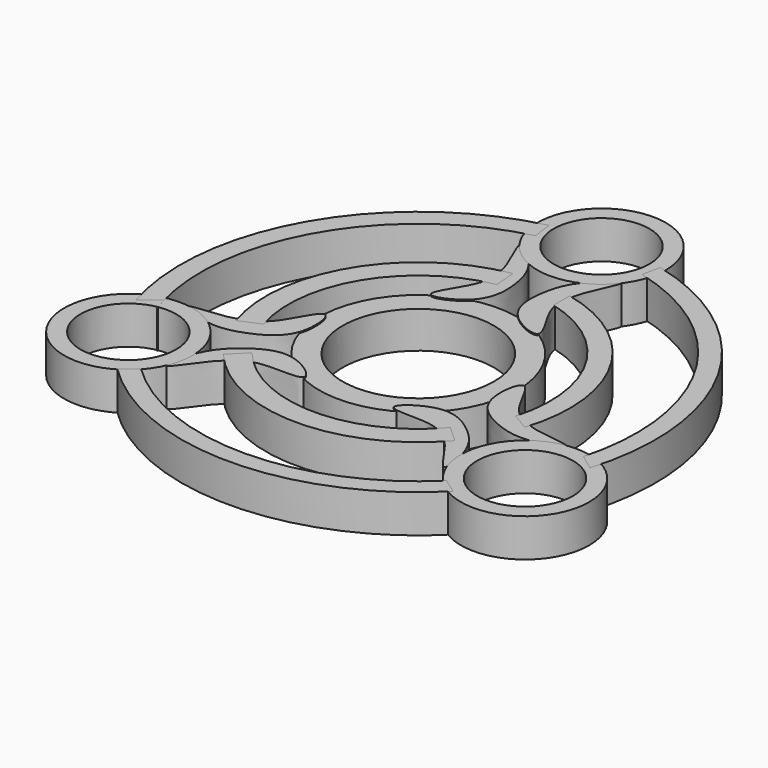
from build123d import *

# Parameters (mm, degrees)
F0_R      = 19.8316168412
F1_DEPTH  = 7.366
F2_R      = 15.1327699345
F3_DEPTH  = 8.89
F4_R      = 12.8405806387
F4_R_2    = 9.5708012392
F5_DEPTH  = 7.62
F7_DEPTH  = 7.62
F8_DEPTH  = 7.62
F10_DEPTH = 7.62
F12_DEPTH = 7.62


# Not quite as in the source:
# - a feature of the source that left no trace in its solid (it failed there, or was rolled back) is left out
# - a feature names something its author has since deleted; it is built from what else it names


with BuildPart() as f1:
    # F0 (on Top) → F1 (new body)
    with BuildSketch(Plane.XY):
        Circle(F0_R)
    extrude(amount=F1_DEPTH)

    # F2 (on Top) → F3 (cut)
    with BuildSketch(Plane.XY):
        Circle(F2_R)
    extrude(amount=F3_DEPTH, mode=Mode.SUBTRACT)


with BuildPart() as f5:
    # F4 (on Top) → F5 (new body)
    with BuildSketch(Plane.XY):
        with Locations((0, 45.8028241992)):
            Circle(F4_R)
        with Locations((0, 45.8028241992)):
            Circle(F4_R_2, mode=Mode.SUBTRACT)
    extrude(amount=F5_DEPTH)


with BuildPart() as f7:
    # F6 (on Top) → F7 (new body)
    with BuildSketch(Plane.XY):
        with BuildLine():
            add(Edge.make_bspline(
                [(-10.1461960003, 38.2656529546), (-10.5971686857, 37.8400995519), (-7.5929666267, 32.2725156605), (-6.9075768698, 28.4550696213), (-6.4560361932, 23.7178665225), (-14.0221319892, 14.0519491431), (-2.2026089144, 18.9490453351), (-2.2410472149, 27.8294457935), (-4.2881589957, 34.1102219148), (-9.6911539418, 38.6950463582), (-10.1461960003, 38.2656529546)],
                knots=[0, 0, 0, 0, 0.1196064646, 0.2243344987, 0.3343048571, 0.4708784974, 0.6015443046, 0.7437811682, 0.8793142609, 1, 1, 1, 1], degree=3))
        make_face()
    extrude(amount=F7_DEPTH)


with BuildPart() as f7b:
    # F6 (on Top) → F7, piece 2 (new body)
    with BuildSketch(Plane.XY):
        with BuildLine():
            add(Edge.make_bspline(
                [(10.1461960003, 38.2656529546), (10.5971686857, 37.8400995519), (7.5929666267, 32.2725156605), (6.9075768698, 28.4550696213), (6.4560361932, 23.7178665225), (14.0221319892, 14.0519491431), (2.2026089144, 18.9490453351), (2.2410472149, 27.8294457935), (4.2881589957, 34.1102219148), (9.6911539418, 38.6950463582), (10.1461960003, 38.2656529546)],
                knots=[0, 0, 0, 0, 0.1196064646, 0.2243344987, 0.3343048571, 0.4708784974, 0.6015443046, 0.7437811682, 0.8793142609, 1, 1, 1, 1], degree=3))
        make_face()
    extrude(amount=F7_DEPTH)


with BuildPart() as f7c:
    # F6 (on Top) → F7, piece 3 (new body)
    with BuildSketch(Plane.XY):
        with BuildLine():
            add(Edge.make_bspline(
                [(38.0458038622, -10.4497247993), (37.9192240951, -9.8427242852), (31.6027522683, -9.488599928), (27.9911987139, -8.074621744), (23.7183170825, -5.9799941528), (19.4420127466, 5.5260471128), (17.4286413404, -7.1083904453), (25.0157130247, -11.7235104937), (31.4389658818, -13.2664421394), (38.1735258277, -11.0622026108), (38.0458038622, -10.4497247993)],
                knots=[0, 0, 0, 0, 0.1196064646, 0.2243344987, 0.3343048571, 0.4708784974, 0.6015443046, 0.7437811682, 0.8793142609, 1, 1, 1, 1], degree=3))
        make_face()
    extrude(amount=F7_DEPTH)


with BuildPart() as f7d:
    # F6 (on Top) → F7, piece 4 (new body)
    with BuildSketch(Plane.XY):
        with BuildLine():
            add(Edge.make_bspline(
                [(27.4250593609, -27.7407906815), (26.8264144307, -27.9023342025), (23.6546544249, -22.4284727808), (20.7605470435, -19.8464588679), (16.9603251319, -16.9823192757), (4.7640505609, -18.3703578085), (15.1230140377, -10.862058899), (22.6698496209, -15.542685191), (26.9502450772, -20.5742883219), (28.0291061914, -27.577789465), (27.4250593609, -27.7407906815)],
                knots=[0, 0, 0, 0, 0.1196064646, 0.2243344987, 0.3343048571, 0.4708784974, 0.6015443046, 0.7437811682, 0.8793142609, 1, 1, 1, 1], degree=3))
        make_face()
    extrude(amount=F7_DEPTH)


with BuildPart() as f7e:
    # F6 (on Top) → F7, piece 5 (new body)
    with BuildSketch(Plane.XY):
        with BuildLine():
            add(Edge.make_bspline(
                [(-27.82798931, -28.063647449), (-27.2341608386, -28.2420845754), (-23.9086099711, -22.860269656), (-20.9425206648, -20.361276337), (-17.0626884028, -17.6059390074), (-4.9106288404, -19.338917014), (-15.0527396932, -11.540182227), (-22.729139541, -16.0051430533), (-27.1503526326, -20.9134717024), (-28.4271762203, -27.8836001869), (-27.82798931, -28.063647449)],
                knots=[0, 0, 0, 0, 0.1196064646, 0.2243344987, 0.3343048571, 0.4708784974, 0.6015443046, 0.7437811682, 0.8793142609, 1, 1, 1, 1], degree=3))
        make_face()
    extrude(amount=F7_DEPTH)


with BuildPart() as f7f:
    # F6 (on Top) → F7, piece 6 (new body)
    with BuildSketch(Plane.XY):
        with BuildLine():
            add(Edge.make_bspline(
                [(-37.9546495422, -10.4786559606), (-37.8109254408, -9.8754848039), (-31.4869568886, -9.700435813), (-27.8367974939, -8.3893333095), (-23.5062939642, -6.416588683), (-18.9057622264, 4.9636956767), (-17.2511076431, -7.722706297), (-24.9658717812, -12.1210473589), (-31.4302550876, -13.48140165), (-38.0996705446, -11.0872698603), (-37.9546495422, -10.4786559606)],
                knots=[0, 0, 0, 0, 0.1196064646, 0.2243344987, 0.3343048571, 0.4708784974, 0.6015443046, 0.7437811682, 0.8793142609, 1, 1, 1, 1], degree=3))
        make_face()
    extrude(amount=F7_DEPTH)


with BuildPart() as f8:
    # F4 (on Top) → F8 (new body)
    with BuildSketch(Plane.XY):
        with Locations((0, 45.8028241992)):
            Circle(F4_R)
        with Locations((0, 45.8028241992)):
            Circle(F4_R_2, mode=Mode.SUBTRACT)
    extrude(amount=F8_DEPTH)


with BuildPart() as f8b:
    # F4 (on Top) → F8, piece 2 (new body)
    with BuildSketch(Plane.XY):
        with Locations((-39.6664093216, -22.9014120996)):
            Circle(F4_R)
        with Locations((-39.6664093216, -22.9014120996)):
            Circle(F4_R_2, mode=Mode.SUBTRACT)
    extrude(amount=F8_DEPTH)


with BuildPart() as f8c:
    # F4 (on Top) → F8, piece 3 (new body)
    with BuildSketch(Plane.XY):
        with Locations((39.6664093216, -22.9014120996)):
            Circle(F4_R)
        with Locations((39.6664093216, -22.9014120996)):
            Circle(F4_R_2, mode=Mode.SUBTRACT)
    extrude(amount=F8_DEPTH)


with BuildPart() as f10:
    # F9 (on Top) → F10 (new body)
    with BuildSketch(Plane.XY):
        with BuildLine():
            Line((-4.7045984098, 25.5188748579), (-5.0730993971, 30.0037506968))
            ThreePointArc((-5.0730993971, 30.0037506968), (-26.0401835333, 15.7438951635), (-28.9256811899, -9.4480876938))
            Line((-28.9256811899, -9.4480876938), (-24.7857067734, -7.6821194962))
            ThreePointArc((-24.7857067734, -7.6821194962), (-22.2035139443, 13.4294522873), (-4.7045984098, 25.5188748579))
        make_face()
    extrude(amount=F10_DEPTH)


with BuildPart() as f10b:
    # F9 (on Top) → F10, piece 2 (new body)
    with BuildSketch(Plane.XY):
        with BuildLine():
            Line((-20.147446543, -16.378859058), (-23.336250335, -19.56766285))
            ThreePointArc((-23.336250335, -19.56766285), (-0.1568800839, -30.4540538804), (23.133416665, -19.8070452747))
            Line((23.133416665, -19.8070452747), (19.8330628805, -16.7581694413))
            ThreePointArc((19.8330628805, -16.7581694413), (-0.2463297861, -25.9639355237), (-20.147446543, -16.378859058))
        make_face()
    extrude(amount=F10_DEPTH)


with BuildPart() as f10c:
    # F9 (on Top) → F10, piece 3 (new body)
    with BuildSketch(Plane.XY):
        with BuildLine():
            Line((25.3654867411, -7.392228581), (28.8441870362, -9.4214677811))
            ThreePointArc((28.8441870362, -9.4214677811), (26.3563547864, 15.036413911), (6.5683197142, 29.6244553884))
            Line((6.5683197142, 29.6244553884), (6.5683197142, 25.5912121076))
            ThreePointArc((6.5683197142, 25.5912121076), (22.9547127753, 13.081824124), (25.3654867411, -7.392228581))
        make_face()
    extrude(amount=F10_DEPTH)


with BuildPart() as f12:
    # F11 (on Top) → F12 (new body)
    with BuildSketch(Plane.XY):
        with BuildLine():
            Line((-10.2911414579, 42.1791858971), (-10.8709242195, 46.2376661599))
            ThreePointArc((-10.8709242195, 46.2376661599), (-41.1584975389, 23.7081598956), (-45.4510247658, -13.7950394358))
            Line((-45.4510247658, -13.7950394358), (-41.9733935129, -11.100700539))
            ThreePointArc((-41.9733935129, -11.100700539), (-37.3173147291, 22.1902982598), (-10.2911414579, 42.1791858971))
        make_face()
    extrude(amount=F12_DEPTH)


with BuildPart() as f12b:
    # F11 (on Top) → F12, piece 2 (new body)
    with BuildSketch(Plane.XY):
        with BuildLine():
            Line((-41.1665908524, -13.7950394358), (-41.9733935129, -11.100700539))
            ThreePointArc((-41.9733935129, -11.100700539), (-41.591815488, -12.4544048375), (-41.1665908524, -13.7950394358))
        make_face()
    extrude(amount=F12_DEPTH)


with BuildPart() as f12c:
    # F11 (on Top) → F12, piece 3 (new body)
    with BuildSketch(Plane.XY):
        with BuildLine():
            Line((-30.2936416119, -31.4532071352), (-33.1925563514, -33.7723381817))
            ThreePointArc((-33.1925563514, -33.7723381817), (0.3088292617, -47.3520986641), (33.6302387387, -33.3365215009))
            Line((33.6302387387, -33.3365215009), (30.5902975902, -31.164766236))
            ThreePointArc((30.5902975902, -31.164766236), (0.206883374, -43.6688236671), (-30.2936416119, -31.4532071352))
        make_face()
    extrude(amount=F12_DEPTH)


with BuildPart() as f12d:
    # F11 (on Top) → F12, piece 4 (new body)
    with BuildSketch(Plane.XY):
        with BuildLine():
            Line((42.1791858971, -11.4507060498), (45.3679896891, -13.7950394358))
            ThreePointArc((45.3679896891, -13.7950394358), (41.3039820945, 23.2924593937), (11.6702090357, 45.9604593377))
            Line((11.6702090357, 45.9604593377), (10.8317642781, 42.3423579245))
            ThreePointArc((10.8317642781, 42.3423579245), (37.7619337767, 22.0054254544), (42.1791858971, -11.4507060498))
        make_face()
    extrude(amount=F12_DEPTH)


solid = Compound([f1.part, f5.part, f7.part, f7b.part, f7c.part, f7d.part, f7e.part, f7f.part, f8.part, f8b.part, f8c.part, f10.part, f10b.part, f10c.part, f12.part, f12b.part, f12c.part, f12d.part])
